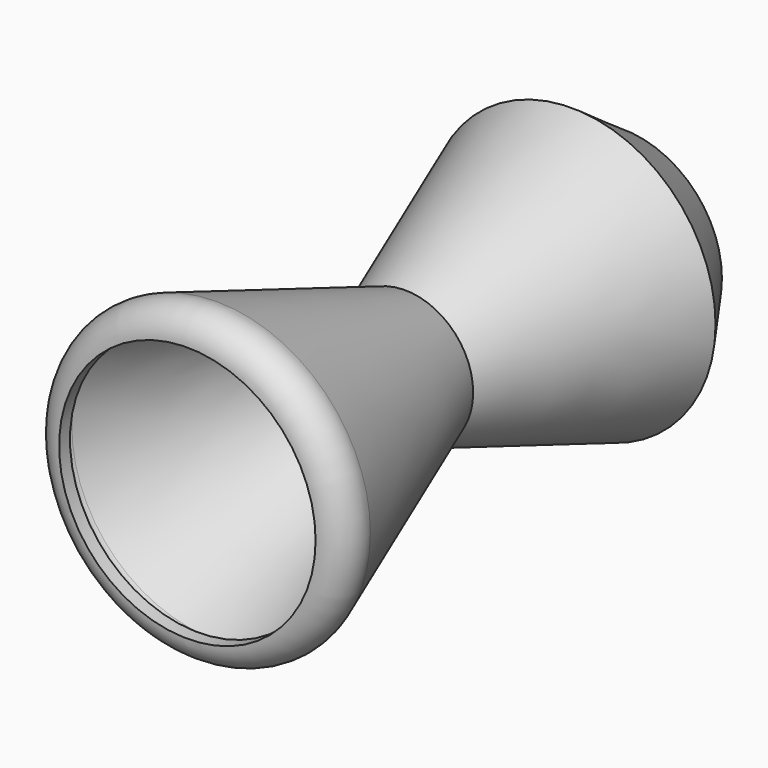
from build123d import *

# Parameters (mm, degrees)
F0_R          = 63.5
F1_DEPTH      = 254
F1_TAPER      = -20
F1_DEPTH_BACK = 254
F1_TAPER_BACK = -20
F2_R          = 25.4
F3_SIZE       = 63.5
F4_T          = -12.7


# Not quite as in the source:
# - a shell that OpenCascade refuses in one call is made with other operations: the cavity is built on its own and cut out


with BuildPart() as f1:
    # F0 (on Front) → F1 (new body, two sides)
    with BuildSketch(Plane.XZ) as f1_sk:
        Circle(F0_R)
    extrude(amount=F1_DEPTH, taper=F1_TAPER)
    extrude(f1_sk.sketch, amount=-F1_DEPTH_BACK, taper=F1_TAPER_BACK)

    # F2
    f2_edges = [f1.edges().sort_by_distance(p)[0] for p in [
        (-155.94844, -254, 0),
    ]]
    fillet(f2_edges, radius=F2_R)

    # F3
    f3_edges = [f1.edges().sort_by_distance(p)[0] for p in [
        (-155.94844, 254, 0),
    ]]
    chamfer(f3_edges, length=F3_SIZE)

    # F4: a shell. OpenCascade refuses it in one call, so the cavity is built on its own and cut out:
    # the body offset inwards by the wall thickness, plus a prism from it out through each open face.
    f4_core = offset(f1.part, amount=F4_T, kind=Kind.INTERSECTION, mode=Mode.PRIVATE)
    f4_exits = [f4_core.faces().sort_by_distance(p)[0] for p in [
        (0, -241.3, 0),
    ]]
    add(f4_core, mode=Mode.SUBTRACT)
    extrude(f4_exits, amount=-F4_T, mode=Mode.SUBTRACT)


solid = f1.part
